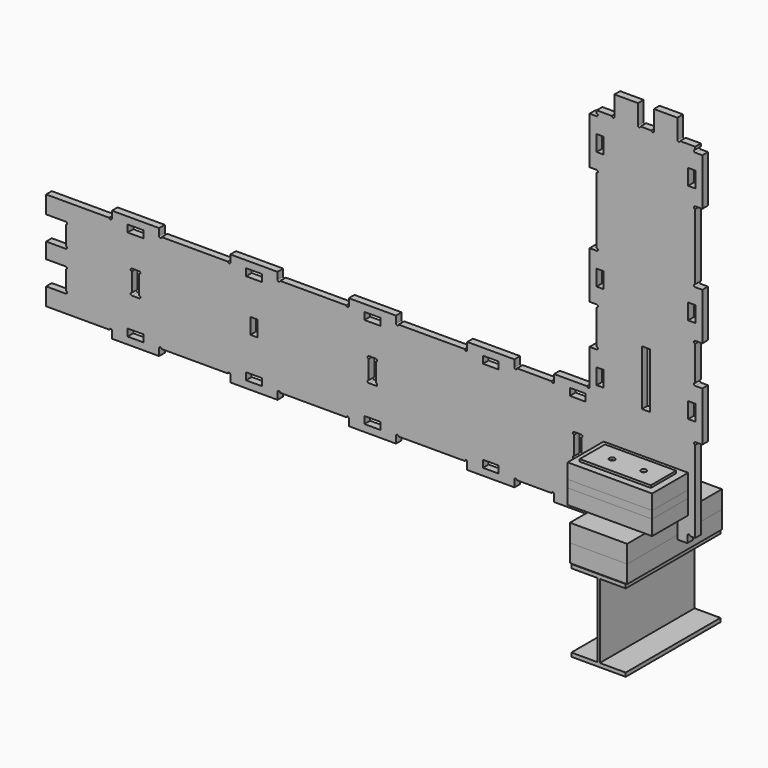
from build123d import *

# Parameters (mm, degrees)
F0_W      = 40
F0_H      = 18
F0_W_2    = 18
F0_H_2    = 40
F0_W_3    = 20
F0_H_3    = 140
F1_DEPTH  = 18
F4_DEPTH  = 150
F5_DEPTH  = 150
F3_W      = 3.15
F3_H      = 187.6
F7_DEPTH  = 150
F6_R      = 8
F8_DEPTH  = 100
F2_W      = 214
F2_H      = 38
F9_DEPTH  = 114
F10_R     = 12.5
F11_DEPTH = 100
F10_W     = 180
F10_H     = 80
F12_DEPTH = 6
F13_R     = 7
F14_DEPTH = 6
F2_H_2    = 19
F15_DEPTH = 114


# Not quite as in the source:
# - ends of sketch curves that miss each other by under 0.0002 mm in the source are joined


with BuildPart() as f1:
    # F0 (on Front) → F1 (new body)
    with BuildSketch(Plane.XZ):
        with BuildLine():
            Line((-425.285768, -73.214369), (-425.285768, 46.285631))
            Line((-425.285768, 46.285631), (-443.035773, 46.285631))
            ThreePointArc((-443.035773, 46.285631), (-446.2933503215, 49.4256374461), (-443.2855219526, 52.8056403944))
            Line((-443.2855219526, 52.8056403944), (-443.285255, 59.590245))
            Line((-443.285255, 59.590245), (-481.765245, 59.590245))
            ThreePointArc((-481.765245, 59.590245), (-485.1457305762, 56.572982213), (-488.2852450833, 59.8402450001))
            Line((-488.2852450833, 59.8402450001), (-488.285245, 109.590245))
            Line((-488.285245, 109.590245), (-547.785245, 109.590245))
            Line((-547.785245, 109.590245), (-547.785245, 59.840245))
            ThreePointArc((-547.785245, 59.840245), (-550.9251258403, 56.5825474923), (-554.3052445294, 59.5902450369))
            Line((-554.3052445294, 59.5902450369), (-581.765245, 59.590245))
            ThreePointArc((-581.765245, 59.590245), (-585.1457305762, 56.572982213), (-588.2852450833, 59.8402450001))
            Line((-588.2852450833, 59.8402450001), (-588.285245, 109.590245))
            Line((-588.285245, 109.590245), (-647.785245, 109.590245))
            Line((-647.785245, 109.590245), (-647.785245, 59.840245))
            ThreePointArc((-647.785245, 59.840245), (-650.9251258403, 56.5825474923), (-654.3052445294, 59.5902450369))
            Line((-654.3052445294, 59.5902450369), (-692.785255, 59.590245))
            Line((-692.785255, 59.590245), (-692.785522, 52.805621))
            ThreePointArc((-692.785522, 52.805621), (-689.7683920315, 49.4250198215), (-693.0357729998, 46.2856311096))
            Line((-693.0357729998, 46.2856311096), (-710.785768, 46.285631))
            Line((-710.785768, 46.285631), (-710.785768, -73.214369))
            Line((-710.785768, -73.214369), (-693.035768, -73.214369))
            ThreePointArc((-693.035768, -73.214369), (-689.7780704923, -76.3542498403), (-692.7857680369, -79.7343685294))
            Line((-692.7857680369, -79.7343685294), (-692.785768, -247.194369))
            ThreePointArc((-692.785768, -247.194369), (-689.768505213, -250.5748545762), (-693.0357680001, -253.7143690833))
            Line((-693.0357680001, -253.7143690833), (-710.785768, -253.714369))
            Line((-710.785768, -253.714369), (-710.785768, -373.214369))
            Line((-710.785768, -373.214369), (-693.035768, -373.214369))
            ThreePointArc((-693.035768, -373.214369), (-689.7780704923, -376.3542498403), (-692.7857680369, -379.7343685294))
            Line((-692.7857680369, -379.7343685294), (-692.785768, -467.194369))
            ThreePointArc((-692.785768, -467.194369), (-689.768505213, -470.5748545762), (-693.0357680001, -473.7143690833))
            Line((-693.0357680001, -473.7143690833), (-710.785768, -473.714369))
            Line((-710.785768, -473.714369), (-710.785768, -563.230661))
            ThreePointArc((-710.785768, -563.230661), (-713.9256488403, -566.4883585077), (-717.3057675294, -563.4806609631))
            Line((-717.3057675294, -563.4806609631), (-800.55138, -563.480661))
            Line((-800.55138, -563.480661), (-800.55138, -581.230661))
            ThreePointArc((-800.55138, -581.230661), (-803.6912608403, -584.4883585077), (-807.0713795294, -581.4806609631))
            Line((-807.0713795294, -581.4806609631), (-894.53138, -581.480661))
            ThreePointArc((-894.53138, -581.480661), (-897.9118655762, -584.497923787), (-901.0513800833, -581.2306609999))
            Line((-901.0513800833, -581.2306609999), (-901.05138, -563.480661))
            Line((-901.05138, -563.480661), (-1020.55138, -563.480661))
            Line((-1020.55138, -563.480661), (-1020.55138, -581.230661))
            ThreePointArc((-1020.55138, -581.230661), (-1023.6912608403, -584.4883585077), (-1027.0713795294, -581.4806609631))
            Line((-1027.0713795294, -581.4806609631), (-1194.53138, -581.480661))
            ThreePointArc((-1194.53138, -581.480661), (-1197.9118655762, -584.497923787), (-1201.0513800833, -581.2306609999))
            Line((-1201.0513800833, -581.2306609999), (-1201.05138, -563.480661))
            Line((-1201.05138, -563.480661), (-1320.55138, -563.480661))
            Line((-1320.55138, -563.480661), (-1320.55138, -581.230661))
            ThreePointArc((-1320.55138, -581.230661), (-1323.6912608403, -584.4883585077), (-1327.0713795294, -581.4806609631))
            Line((-1327.0713795294, -581.4806609631), (-1494.53138, -581.480661))
            ThreePointArc((-1494.53138, -581.480661), (-1497.9118655762, -584.497923787), (-1501.0513800833, -581.2306609999))
            Line((-1501.0513800833, -581.2306609999), (-1501.05138, -563.480661))
            Line((-1501.05138, -563.480661), (-1620.55138, -563.480661))
            Line((-1620.55138, -563.480661), (-1620.55138, -581.230661))
            ThreePointArc((-1620.55138, -581.230661), (-1623.6912608403, -584.4883585077), (-1627.0713795294, -581.4806609631))
            Line((-1627.0713795294, -581.4806609631), (-1794.53138, -581.480661))
            ThreePointArc((-1794.53138, -581.480661), (-1797.9118655762, -584.497923787), (-1801.0513800833, -581.2306609999))
            Line((-1801.0513800833, -581.2306609999), (-1801.05138, -563.480661))
            Line((-1801.05138, -563.480661), (-1920.55138, -563.480661))
            Line((-1920.55138, -563.480661), (-1920.55138, -581.230661))
            ThreePointArc((-1920.55138, -581.230661), (-1923.6912608403, -584.4883585077), (-1927.0713795294, -581.4806609631))
            Line((-1927.0713795294, -581.4806609631), (-2087.246461, -581.480661))
            Line((-2087.246461, -581.480661), (-2087.246461, -625.980661))
            Line((-2087.246461, -625.980661), (-2037.496461, -625.980661))
            ThreePointArc((-2037.496461, -625.980661), (-2034.2387634923, -629.1205418403), (-2037.2464610369, -632.5006605294))
            Line((-2037.2464610369, -632.5006605294), (-2037.246461, -679.960661))
            ThreePointArc((-2037.246461, -679.960661), (-2034.229198213, -683.3411465762), (-2037.4964610001, -686.4806610833))
            Line((-2037.4964610001, -686.4806610833), (-2087.246461, -686.480661))
            Line((-2087.246461, -686.480661), (-2087.246461, -725.980661))
            Line((-2087.246461, -725.980661), (-2037.496461, -725.980661))
            ThreePointArc((-2037.496461, -725.980661), (-2034.2387634923, -729.1205418403), (-2037.2464610369, -732.5006605294))
            Line((-2037.2464610369, -732.5006605294), (-2037.246461, -779.960661))
            ThreePointArc((-2037.246461, -779.960661), (-2034.229198213, -783.3411465762), (-2037.4964610001, -786.4806610833))
            Line((-2037.4964610001, -786.4806610833), (-2087.246461, -786.480661))
            Line((-2087.246461, -786.480661), (-2087.246461, -830.980661))
            Line((-2087.246461, -830.980661), (-1927.07138, -830.980661))
            ThreePointArc((-1927.07138, -830.980661), (-1923.6908944238, -827.963398213), (-1920.5513799167, -831.2306610001))
            Line((-1920.5513799167, -831.2306610001), (-1920.55138, -848.980661))
            Line((-1920.55138, -848.980661), (-1801.05138, -848.980661))
            Line((-1801.05138, -848.980661), (-1801.05138, -831.230661))
            ThreePointArc((-1801.05138, -831.230661), (-1797.9114991597, -827.9729634923), (-1794.5313804706, -830.9806610369))
            Line((-1794.5313804706, -830.9806610369), (-1627.07138, -830.980661))
            ThreePointArc((-1627.07138, -830.980661), (-1623.6908944238, -827.963398213), (-1620.5513799167, -831.2306610001))
            Line((-1620.5513799167, -831.2306610001), (-1620.55138, -848.980661))
            Line((-1620.55138, -848.980661), (-1501.05138, -848.980661))
            Line((-1501.05138, -848.980661), (-1501.05138, -831.230661))
            ThreePointArc((-1501.05138, -831.230661), (-1497.9114991597, -827.9729634923), (-1494.5313804706, -830.9806610369))
            Line((-1494.5313804706, -830.9806610369), (-1327.07138, -830.980661))
            ThreePointArc((-1327.07138, -830.980661), (-1323.6908944238, -827.963398213), (-1320.5513799168, -831.2306610001))
            Line((-1320.5513799168, -831.2306610001), (-1320.55138, -848.980661))
            Line((-1320.55138, -848.980661), (-1201.05138, -848.980661))
            Line((-1201.05138, -848.980661), (-1201.05138, -831.230661))
            ThreePointArc((-1201.05138, -831.230661), (-1197.9114991597, -827.9729634923), (-1194.5313804706, -830.9806610369))
            Line((-1194.5313804706, -830.9806610369), (-1027.07138, -830.980661))
            ThreePointArc((-1027.07138, -830.980661), (-1023.6908944238, -827.963398213), (-1020.5513799167, -831.2306610001))
            Line((-1020.5513799167, -831.2306610001), (-1020.55138, -848.980661))
            Line((-1020.55138, -848.980661), (-901.05138, -848.980661))
            Line((-901.05138, -848.980661), (-901.05138, -831.230661))
            ThreePointArc((-901.05138, -831.230661), (-897.9114991597, -827.9729634923), (-894.5313804706, -830.9806610369))
            Line((-894.5313804706, -830.9806610369), (-807.07138, -830.980661))
            ThreePointArc((-807.07138, -830.980661), (-803.6908944238, -827.963398213), (-800.5513799167, -831.2306610001))
            Line((-800.5513799167, -831.2306610001), (-800.55138, -848.980661))
            Line((-800.55138, -848.980661), (-681.05138, -848.980661))
            Line((-681.05138, -848.980661), (-681.05138, -831.230661))
            ThreePointArc((-681.05138, -831.230661), (-677.9114991597, -827.9729634923), (-674.5313804706, -830.9806610369))
            Line((-674.5313804706, -830.9806610369), (-648.285452, -830.980661))
            Line((-648.285452, -830.980661), (-648.285452, -787.500661))
            ThreePointArc((-648.285452, -787.500661), (-651.302714787, -784.1201754238), (-648.0354519999, -780.9806609167))
            Line((-648.0354519999, -780.9806609167), (-488.035452, -780.980661))
            ThreePointArc((-488.035452, -780.980661), (-484.7777544923, -784.1205418403), (-487.7854520369, -787.5006605294))
            Line((-487.7854520369, -787.5006605294), (-487.785452, -830.980661))
            Line((-487.785452, -830.980661), (-463.285452, -830.980661))
            Line((-463.285452, -830.980661), (-463.285452, -813.230661))
            ThreePointArc((-463.285452, -813.230661), (-460.1455711597, -809.9729634923), (-456.7654524706, -812.9806610369))
            Line((-456.7654524706, -812.9806610369), (-443.285453, -812.980661))
            Line((-443.285453, -812.980661), (-443.285759, -605.505391))
            ThreePointArc((-443.285759, -605.505391), (-446.3030269605, -602.1249089509), (-443.0357679999, -598.9853899106))
            Line((-443.0357679999, -598.9853899106), (-425.285768, -598.98539))
            Line((-425.285768, -598.98539), (-425.285768, -473.714369))
            Line((-425.285768, -473.714369), (-443.035768, -473.714369))
            ThreePointArc((-443.035768, -473.714369), (-446.2934655077, -470.5744881597), (-443.2857679631, -467.1943694706))
            Line((-443.2857679631, -467.1943694706), (-443.285768, -379.734369))
            ThreePointArc((-443.285768, -379.734369), (-446.303030787, -376.3538834238), (-443.0357679999, -373.2143689167))
            Line((-443.0357679999, -373.2143689167), (-425.285768, -373.214369))
            Line((-425.285768, -373.214369), (-425.285768, -253.714369))
            Line((-425.285768, -253.714369), (-443.035768, -253.714369))
            ThreePointArc((-443.035768, -253.714369), (-446.2934655077, -250.5744881597), (-443.2857679631, -247.1943694706))
            Line((-443.2857679631, -247.1943694706), (-443.285768, -79.734369))
            ThreePointArc((-443.285768, -79.734369), (-446.303030787, -76.3538834238), (-443.0357679999, -73.2143689167))
            Line((-443.0357679999, -73.2143689167), (-425.285768, -73.214369))
        make_face()
        with Locations((-1860.80138, -822.230661)):
            Rectangle(F0_W, F0_H, mode=Mode.SUBTRACT)
        with BuildLine():
            ThreePointArc((-1870.0513799891, -682.4982378555), (-1873.0662218614, -679.1190115833), (-1869.8013799991, -675.9806602124))
            Line((-1869.8013799991, -675.9806602124), (-1851.80138, -675.980661))
            ThreePointArc((-1851.80138, -675.980661), (-1848.5436893491, -679.1192866301), (-1851.5513799547, -682.4982385807))
            Line((-1851.5513799547, -682.4982385807), (-1851.55138, -729.963084))
            ThreePointArc((-1851.55138, -729.963084), (-1848.5365381386, -733.3423104167), (-1851.8013800009, -736.4806617876))
            Line((-1851.8013800009, -736.4806617876), (-1869.80138, -736.480661))
            ThreePointArc((-1869.80138, -736.480661), (-1873.0590706509, -733.3420353699), (-1870.0513800453, -729.9630834193))
            Line((-1870.0513800453, -729.9630834193), (-1870.0513799891, -682.4982378555))
        make_face(mode=Mode.SUBTRACT)
        with Locations((-1560.80138, -822.230661)):
            Rectangle(F0_W, F0_H, mode=Mode.SUBTRACT)
        with Locations((-1260.80138, -822.230661)):
            Rectangle(F0_W, F0_H, mode=Mode.SUBTRACT)
        with Locations((-1560.80138, -706.230661)):
            Rectangle(F0_W_2, F0_H_2, mode=Mode.SUBTRACT)
        with BuildLine():
            ThreePointArc((-1270.0513799891, -682.4982378555), (-1273.0662218614, -679.1190115833), (-1269.8013799991, -675.9806602124))
            Line((-1269.8013799991, -675.9806602124), (-1251.80138, -675.980661))
            ThreePointArc((-1251.80138, -675.980661), (-1248.5436893491, -679.1192866301), (-1251.5513799547, -682.4982385807))
            Line((-1251.5513799547, -682.4982385807), (-1251.55138, -729.963084))
            ThreePointArc((-1251.55138, -729.963084), (-1248.5365381386, -733.3423104167), (-1251.8013800009, -736.4806617876))
            Line((-1251.8013800009, -736.4806617876), (-1269.80138, -736.480661))
            ThreePointArc((-1269.80138, -736.480661), (-1273.0590706509, -733.3420353699), (-1270.0513800453, -729.9630834193))
            Line((-1270.0513800453, -729.9630834193), (-1270.0513799891, -682.4982378555))
        make_face(mode=Mode.SUBTRACT)
        with Locations((-1860.80138, -590.230661)):
            Rectangle(F0_W, F0_H, mode=Mode.SUBTRACT)
        with Locations((-1560.80138, -590.230661)):
            Rectangle(F0_W, F0_H, mode=Mode.SUBTRACT)
        with Locations((-1260.80138, -590.230661)):
            Rectangle(F0_W, F0_H, mode=Mode.SUBTRACT)
        with Locations((-960.80138, -822.230661)):
            Rectangle(F0_W, F0_H, mode=Mode.SUBTRACT)
        with Locations((-740.80138, -822.230661)):
            Rectangle(F0_W, F0_H, mode=Mode.SUBTRACT)
        with BuildLine():
            ThreePointArc((-750.0513799891, -682.4982378555), (-753.0662218614, -679.1190115833), (-749.8013799991, -675.9806602124))
            Line((-749.8013799991, -675.9806602124), (-731.80138, -675.980661))
            ThreePointArc((-731.80138, -675.980661), (-728.5436893491, -679.1192866301), (-731.5513799547, -682.4982385807))
            Line((-731.5513799547, -682.4982385807), (-731.55138, -729.963084))
            ThreePointArc((-731.55138, -729.963084), (-728.5365381386, -733.3423104167), (-731.8013800009, -736.4806617876))
            Line((-731.8013800009, -736.4806617876), (-749.80138, -736.480661))
            ThreePointArc((-749.80138, -736.480661), (-753.0590706509, -733.3420353699), (-750.0513800453, -729.9630834193))
            Line((-750.0513800453, -729.9630834193), (-750.0513799891, -682.4982378555))
        make_face(mode=Mode.SUBTRACT)
        with Locations((-960.80138, -590.230661)):
            Rectangle(F0_W, F0_H, mode=Mode.SUBTRACT)
        with Locations((-740.80138, -590.230661)):
            Rectangle(F0_W, F0_H, mode=Mode.SUBTRACT)
        with Locations((-684.035768, -533.464369)):
            Rectangle(F0_W_2, F0_H_2, mode=Mode.SUBTRACT)
        with Locations((-568.035452, -499.230661)):
            Rectangle(F0_W_3, F0_H_3, mode=Mode.SUBTRACT)
        with Locations((-452.035768, -533.464369)):
            Rectangle(F0_W_2, F0_H_2, mode=Mode.SUBTRACT)
        with Locations((-684.035768, -313.464369)):
            Rectangle(F0_W_2, F0_H_2, mode=Mode.SUBTRACT)
        with Locations((-452.035768, -313.464369)):
            Rectangle(F0_W_2, F0_H_2, mode=Mode.SUBTRACT)
        with Locations((-684.035768, -13.464369)):
            Rectangle(F0_W_2, F0_H_2, mode=Mode.SUBTRACT)
        with Locations((-452.035768, -13.464369)):
            Rectangle(F0_W_2, F0_H_2, mode=Mode.SUBTRACT)
    extrude(amount=F1_DEPTH)


with BuildPart() as f4:
    # F3 (on face) → F4 (new body, symmetric)
    with BuildSketch(Plane.XZ.offset(18)):
        Polygon((-495.535452, -781.980661), (-640.535452, -781.980661), (-640.535452, -826.980661), (-568.035452, -826.980661), (-495.535452, -826.980661), align=None)
    extrude(amount=F4_DEPTH, both=True)


with BuildPart() as f5:
    # F3 (on face) → F5 (new body, symmetric)
    with BuildSketch(Plane.XZ.offset(18)):
        Polygon((-568.035452, -826.980661), (-640.535452, -826.980661), (-640.535452, -871.980661), (-636.8328928947, -871.980661), (-568.035452, -871.980661), align=None)
        Polygon((-495.535452, -871.980661), (-495.535452, -826.980661), (-568.035452, -826.980661), (-568.035452, -871.980661), (-499.2380111051, -871.980661), align=None)
    extrude(amount=F5_DEPTH, both=True)


with BuildPart() as f7:
    # F3 (on face) → F7 (new body, symmetric)
    with BuildSketch(Plane.XZ.offset(18)):
        Polygon((-499.2380111051, -872.980661), (-568.035452, -872.980661), (-568.035452, -882.580661), (-564.885452, -882.580661), (-499.2380111051, -882.580661), align=None)
        Polygon((-568.035452, -882.580661), (-568.035452, -872.980661), (-636.8328928947, -872.980661), (-636.8328928947, -882.580661), (-571.185452, -882.580661), align=None)
        with Locations((-566.460452, -976.380661)):
            Rectangle(F3_W, F3_H)
        with Locations((-569.610452, -976.380661)):
            Rectangle(F3_W, F3_H)
        Polygon((-564.885452, -1070.180661), (-568.035452, -1070.180661), (-568.035452, -1079.780661), (-499.2380111051, -1079.780661), (-499.2380111051, -1070.180661), align=None)
        Polygon((-568.035452, -1079.780661), (-568.035452, -1070.180661), (-571.185452, -1070.180661), (-636.8328928947, -1070.180661), (-636.8328928947, -1079.780661), align=None)
    extrude(amount=F7_DEPTH, both=True)


with BuildPart() as f8_tool:
    # F6 (on face) → F8 (new body, symmetric)
    with BuildSketch(Plane(origin=(0, 0, -871.980661), x_dir=(1, 0, 0), z_dir=(0, 0, -1))):
        with Locations((-608.035452, 75)):
            Circle(F6_R)
        with Locations((-528.035452, 75)):
            Circle(F6_R)
    extrude(amount=F8_DEPTH, both=True)


with BuildPart() as f4_1:
    add(f4.part)

    # F8: cut by f8_tool
    add(f8_tool.part, mode=Mode.SUBTRACT)


with BuildPart() as f5_1:
    add(f5.part)

    # F8: cut by f8_tool
    add(f8_tool.part, mode=Mode.SUBTRACT)


with BuildPart() as f7_1:
    add(f7.part)

    # F8: cut by f8_tool
    add(f8_tool.part, mode=Mode.SUBTRACT)


with BuildPart() as f9:
    # F2 (on face) → F9 (new body)
    with BuildSketch(Plane.XZ.offset(18)):
        with Locations((-568.035768, -692.230661)):
            Rectangle(F2_W, F2_H)
    extrude(amount=F9_DEPTH)


with BuildPart() as f9b:
    # F2 (on face) → F9, piece 2 (new body)
    with BuildSketch(Plane.XZ.offset(18)):
        with Locations((-568.035768, -749.230661)):
            Rectangle(F2_W, F2_H)
    extrude(amount=F9_DEPTH)


with BuildPart() as f11_tool:
    # F10 (on face) → F11 (new body)
    with BuildSketch(Plane.XY.offset(-673.230661)):
        with Locations((-608.035768, -75)):
            Circle(F10_R)
        with Locations((-528.035768, -75)):
            Circle(F10_R)
    extrude(amount=-F11_DEPTH)


with BuildPart() as f9_1:
    add(f9.part)

    # F11: cut by f11_tool
    add(f11_tool.part, mode=Mode.SUBTRACT)


with BuildPart() as f9b_1:
    add(f9b.part)

    # F11: cut by f11_tool
    add(f11_tool.part, mode=Mode.SUBTRACT)


with BuildPart() as f12:
    # F10 (on face) → F12 (new body)
    with BuildSketch(Plane.XY.offset(-673.230661)):
        with Locations((-568.035768, -75)):
            Rectangle(F10_W, F10_H)
        with Locations((-608.035768, -75)):
            Circle(F10_R, mode=Mode.SUBTRACT)
        with Locations((-528.035768, -75)):
            Circle(F10_R, mode=Mode.SUBTRACT)
        with Locations((-608.035768, -75)):
            Circle(F10_R)
        with Locations((-528.035768, -75)):
            Circle(F10_R)
    extrude(amount=F12_DEPTH)

    # F13 (on face) → F14 (cut)
    with BuildSketch(Plane.XY.offset(-667.230661)):
        with Locations((-608.035768, -75)):
            Circle(F13_R)
        with Locations((-528.035768, -75)):
            Circle(F13_R)
    extrude(amount=-F14_DEPTH, mode=Mode.SUBTRACT)


with BuildPart() as f15:
    # F2 (on face) → F15 (new body)
    with BuildSketch(Plane.XZ.offset(18)):
        with Locations((-568.035768, -720.730661)):
            Rectangle(F2_W, F2_H_2)
    extrude(amount=F15_DEPTH)


solid = Compound([f1.part, f4_1.part, f5_1.part, f7_1.part, f9_1.part, f9b_1.part, f12.part, f15.part])
